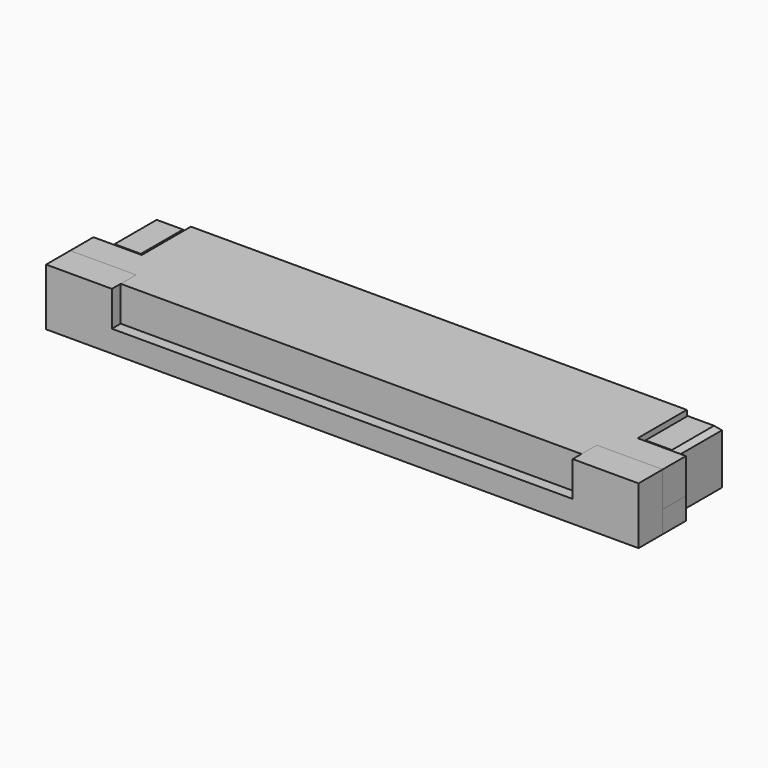
from build123d import *

# Parameters (mm, degrees)
F1_DEPTH   = 1
F2_DEPTH   = 2.6
F0_W       = 21
F0_H       = 0.5
F3_DEPTH   = 1
F5_DEPTH   = 1.6
F0_W_2     = 1.6
F0_H_2     = 2.8
F6_DEPTH   = 2.5
F0_W_3     = 0.6
F0_H_3     = 1.37
F7_DEPTH   = 0.3
F8_SIZE    = 0.2
F8_2_SIZE  = 0.2
F8_3_SIZE  = 0.2
F8_4_SIZE  = 0.2
F8_5_SIZE  = 0.2
F8_6_SIZE  = 0.2
F8_7_SIZE  = 0.2
F8_8_SIZE  = 0.2
F8_9_SIZE  = 0.2
F8_10_SIZE = 0.2
F8_11_SIZE = 0.2
F8_12_SIZE = 0.2
F8_13_SIZE = 0.2
F8_14_SIZE = 0.2
F8_15_SIZE = 0.2
F8_16_SIZE = 0.2
F8_17_SIZE = 0.2
F8_18_SIZE = 0.2
F8_19_SIZE = 0.2
F8_20_SIZE = 0.2
F9_SIZE    = 0.2
F9_2_SIZE  = 0.2


with BuildPart() as f1:
    # F0 (on Top) → F1 (new body)
    with BuildSketch(Plane.XY):
        Polygon((-9.8, 2.75), (-11.3, 2.75), (-11.3, -0.05), (-12.9, -0.05), (-13.5, -0.05), (-13.5, -1.375), (-10.5, -1.375), (-10.5, -2.25), (10.5, -2.25), (10.5, -1.375), (13.5, -1.375), (13.5, -0.05), (12.9, -0.05), (11.3, -0.05), (11.3, 2.75), (9.8, 2.75), (9.2, 2.75), (8.8, 2.75), (8.2, 2.75), (7.8, 2.75), (7.2, 2.75), (6.8, 2.75), (6.2, 2.75), (5.8, 2.75), (5.2, 2.75), (4.8, 2.75), (4.2, 2.75), (3.8, 2.75), (3.2, 2.75), (2.8, 2.75), (2.2, 2.75), (1.8, 2.75), (1.2, 2.75), (0.8, 2.75), (0.2, 2.75), (-0.2, 2.75), (-0.8, 2.75), (-1.2, 2.75), (-1.8, 2.75), (-2.2, 2.75), (-2.8, 2.75), (-3.2, 2.75), (-3.8, 2.75), (-4.2, 2.75), (-4.8, 2.75), (-5.2, 2.75), (-5.8, 2.75), (-6.2, 2.75), (-6.8, 2.75), (-7.2, 2.75), (-7.8, 2.75), (-8.2, 2.75), (-8.8, 2.75), (-9.2, 2.75), align=None)
    extrude(amount=F1_DEPTH)


with BuildPart() as f2:
    # F0 (on Top) → F2 (new body)
    with BuildSketch(Plane.XY):
        Polygon((-10.5, -1.375), (-13.5, -1.375), (-13.5, -2.75), (-10.5, -2.75), (-10.5, -2.25), align=None)
    extrude(amount=F2_DEPTH)



with BuildPart() as f2b:
    # F0 (on Top) → F2, piece 2 (new body)
    with BuildSketch(Plane.XY):
        Polygon((10.5, -2.25), (10.5, -2.75), (13.5, -2.75), (13.5, -1.375), (10.5, -1.375), align=None)
    extrude(amount=F2_DEPTH)


with BuildPart() as f2_1:
    add(f2.part)

    add(f2b.part)  # F3 merges F2b
    # F0 (on Top) → F3 (join)
    with BuildSketch(Plane.XY):
        with Locations((0, -2.5)):
            Rectangle(F0_W, F0_H)
    extrude(amount=F3_DEPTH)


with BuildPart() as f5:
    # F5 (new): a face of the model
    f5_faces = [f1.part.faces().sort_by_distance(p)[0] for p in [
        (0, 0.2268042664, 1),
    ]]
    extrude(f5_faces, amount=F5_DEPTH)


with BuildPart() as f6:
    # F0 (on Top) → F6 (new body)
    with BuildSketch(Plane.XY):
        with Locations((-12.1, 1.35)):
            Rectangle(F0_W_2, F0_H_2)
    extrude(amount=F6_DEPTH)

    # F9
    f9_edges = [f6.edges().sort_by_distance(p)[0] for p in [
        (-12.1, 2.75, 2.5),
        (-12.9, 1.35, 2.5),
        (-11.3, 1.35, 2.5),
        (-12.1, -0.05, 2.5),
    ]]
    chamfer(f9_edges, length=F9_SIZE)


with BuildPart() as f6b:
    # F0 (on Top) → F6, piece 2 (new body)
    with BuildSketch(Plane.XY):
        with Locations((12.1, 1.35)):
            Rectangle(F0_W_2, F0_H_2)
    extrude(amount=F6_DEPTH)

    # F9#2
    f9_2_edges = [f6b.edges().sort_by_distance(p)[0] for p in [
        (12.1, 2.75, 2.5),
        (12.9, 1.35, 2.5),
        (11.3, 1.35, 2.5),
        (12.1, -0.05, 2.5),
    ]]
    chamfer(f9_2_edges, length=F9_2_SIZE)


with BuildPart() as f7:
    # F0 (on Top) → F7 (new body)
    with BuildSketch(Plane.XY):
        with Locations((-9.5, 3.435)):
            Rectangle(F0_W_3, F0_H_3)
    extrude(amount=F7_DEPTH)

    # F8
    f8_edges = [f7.edges().sort_by_distance(p)[0] for p in [
        (-9.5, 4.12, 0.3),
    ]]
    chamfer(f8_edges, length=F8_SIZE)


with BuildPart() as f7b:
    # F0 (on Top) → F7, piece 2 (new body)
    with BuildSketch(Plane.XY):
        with Locations((-8.5, 3.435)):
            Rectangle(F0_W_3, F0_H_3)
    extrude(amount=F7_DEPTH)

    # F8#2
    f8_2_edges = [f7b.edges().sort_by_distance(p)[0] for p in [
        (-8.5, 4.12, 0.3),
    ]]
    chamfer(f8_2_edges, length=F8_2_SIZE)


with BuildPart() as f7c:
    # F0 (on Top) → F7, piece 3 (new body)
    with BuildSketch(Plane.XY):
        with Locations((-7.5, 3.435)):
            Rectangle(F0_W_3, F0_H_3)
    extrude(amount=F7_DEPTH)

    # F8#3
    f8_3_edges = [f7c.edges().sort_by_distance(p)[0] for p in [
        (-7.5, 4.12, 0.3),
    ]]
    chamfer(f8_3_edges, length=F8_3_SIZE)


with BuildPart() as f7d:
    # F0 (on Top) → F7, piece 4 (new body)
    with BuildSketch(Plane.XY):
        with Locations((-6.5, 3.435)):
            Rectangle(F0_W_3, F0_H_3)
    extrude(amount=F7_DEPTH)

    # F8#4
    f8_4_edges = [f7d.edges().sort_by_distance(p)[0] for p in [
        (-6.5, 4.12, 0.3),
    ]]
    chamfer(f8_4_edges, length=F8_4_SIZE)


with BuildPart() as f7e:
    # F0 (on Top) → F7, piece 5 (new body)
    with BuildSketch(Plane.XY):
        with Locations((-5.5, 3.435)):
            Rectangle(F0_W_3, F0_H_3)
    extrude(amount=F7_DEPTH)

    # F8#5
    f8_5_edges = [f7e.edges().sort_by_distance(p)[0] for p in [
        (-5.5, 4.12, 0.3),
    ]]
    chamfer(f8_5_edges, length=F8_5_SIZE)


with BuildPart() as f7f:
    # F0 (on Top) → F7, piece 6 (new body)
    with BuildSketch(Plane.XY):
        with Locations((-4.5, 3.435)):
            Rectangle(F0_W_3, F0_H_3)
    extrude(amount=F7_DEPTH)

    # F8#6
    f8_6_edges = [f7f.edges().sort_by_distance(p)[0] for p in [
        (-4.5, 4.12, 0.3),
    ]]
    chamfer(f8_6_edges, length=F8_6_SIZE)


with BuildPart() as f7g:
    # F0 (on Top) → F7, piece 7 (new body)
    with BuildSketch(Plane.XY):
        with Locations((-3.5, 3.435)):
            Rectangle(F0_W_3, F0_H_3)
    extrude(amount=F7_DEPTH)

    # F8#7
    f8_7_edges = [f7g.edges().sort_by_distance(p)[0] for p in [
        (-3.5, 4.12, 0.3),
    ]]
    chamfer(f8_7_edges, length=F8_7_SIZE)


with BuildPart() as f7h:
    # F0 (on Top) → F7, piece 8 (new body)
    with BuildSketch(Plane.XY):
        with Locations((-2.5, 3.435)):
            Rectangle(F0_W_3, F0_H_3)
    extrude(amount=F7_DEPTH)

    # F8#8
    f8_8_edges = [f7h.edges().sort_by_distance(p)[0] for p in [
        (-2.5, 4.12, 0.3),
    ]]
    chamfer(f8_8_edges, length=F8_8_SIZE)


with BuildPart() as f7i:
    # F0 (on Top) → F7, piece 9 (new body)
    with BuildSketch(Plane.XY):
        with Locations((-1.5, 3.435)):
            Rectangle(F0_W_3, F0_H_3)
    extrude(amount=F7_DEPTH)

    # F8#9
    f8_9_edges = [f7i.edges().sort_by_distance(p)[0] for p in [
        (-1.5, 4.12, 0.3),
    ]]
    chamfer(f8_9_edges, length=F8_9_SIZE)


with BuildPart() as f7j:
    # F0 (on Top) → F7, piece 10 (new body)
    with BuildSketch(Plane.XY):
        with Locations((-0.5, 3.435)):
            Rectangle(F0_W_3, F0_H_3)
    extrude(amount=F7_DEPTH)

    # F8#10
    f8_10_edges = [f7j.edges().sort_by_distance(p)[0] for p in [
        (-0.5, 4.12, 0.3),
    ]]
    chamfer(f8_10_edges, length=F8_10_SIZE)


with BuildPart() as f7k:
    # F0 (on Top) → F7, piece 11 (new body)
    with BuildSketch(Plane.XY):
        with Locations((0.5, 3.435)):
            Rectangle(F0_W_3, F0_H_3)
    extrude(amount=F7_DEPTH)

    # F8#11
    f8_11_edges = [f7k.edges().sort_by_distance(p)[0] for p in [
        (0.5, 4.12, 0.3),
    ]]
    chamfer(f8_11_edges, length=F8_11_SIZE)


with BuildPart() as f7l:
    # F0 (on Top) → F7, piece 12 (new body)
    with BuildSketch(Plane.XY):
        with Locations((1.5, 3.435)):
            Rectangle(F0_W_3, F0_H_3)
    extrude(amount=F7_DEPTH)

    # F8#12
    f8_12_edges = [f7l.edges().sort_by_distance(p)[0] for p in [
        (1.5, 4.12, 0.3),
    ]]
    chamfer(f8_12_edges, length=F8_12_SIZE)


with BuildPart() as f7m:
    # F0 (on Top) → F7, piece 13 (new body)
    with BuildSketch(Plane.XY):
        with Locations((2.5, 3.435)):
            Rectangle(F0_W_3, F0_H_3)
    extrude(amount=F7_DEPTH)

    # F8#13
    f8_13_edges = [f7m.edges().sort_by_distance(p)[0] for p in [
        (2.5, 4.12, 0.3),
    ]]
    chamfer(f8_13_edges, length=F8_13_SIZE)


with BuildPart() as f7n:
    # F0 (on Top) → F7, piece 14 (new body)
    with BuildSketch(Plane.XY):
        with Locations((3.5, 3.435)):
            Rectangle(F0_W_3, F0_H_3)
    extrude(amount=F7_DEPTH)

    # F8#14
    f8_14_edges = [f7n.edges().sort_by_distance(p)[0] for p in [
        (3.5, 4.12, 0.3),
    ]]
    chamfer(f8_14_edges, length=F8_14_SIZE)


with BuildPart() as f7o:
    # F0 (on Top) → F7, piece 15 (new body)
    with BuildSketch(Plane.XY):
        with Locations((4.5, 3.435)):
            Rectangle(F0_W_3, F0_H_3)
    extrude(amount=F7_DEPTH)

    # F8#15
    f8_15_edges = [f7o.edges().sort_by_distance(p)[0] for p in [
        (4.5, 4.12, 0.3),
    ]]
    chamfer(f8_15_edges, length=F8_15_SIZE)


with BuildPart() as f7p:
    # F0 (on Top) → F7, piece 16 (new body)
    with BuildSketch(Plane.XY):
        with Locations((5.5, 3.435)):
            Rectangle(F0_W_3, F0_H_3)
    extrude(amount=F7_DEPTH)

    # F8#16
    f8_16_edges = [f7p.edges().sort_by_distance(p)[0] for p in [
        (5.5, 4.12, 0.3),
    ]]
    chamfer(f8_16_edges, length=F8_16_SIZE)


with BuildPart() as f7q:
    # F0 (on Top) → F7, piece 17 (new body)
    with BuildSketch(Plane.XY):
        with Locations((6.5, 3.435)):
            Rectangle(F0_W_3, F0_H_3)
    extrude(amount=F7_DEPTH)

    # F8#17
    f8_17_edges = [f7q.edges().sort_by_distance(p)[0] for p in [
        (6.5, 4.12, 0.3),
    ]]
    chamfer(f8_17_edges, length=F8_17_SIZE)


with BuildPart() as f7r:
    # F0 (on Top) → F7, piece 18 (new body)
    with BuildSketch(Plane.XY):
        with Locations((7.5, 3.435)):
            Rectangle(F0_W_3, F0_H_3)
    extrude(amount=F7_DEPTH)

    # F8#18
    f8_18_edges = [f7r.edges().sort_by_distance(p)[0] for p in [
        (7.5, 4.12, 0.3),
    ]]
    chamfer(f8_18_edges, length=F8_18_SIZE)


with BuildPart() as f7s:
    # F0 (on Top) → F7, piece 19 (new body)
    with BuildSketch(Plane.XY):
        with Locations((8.5, 3.435)):
            Rectangle(F0_W_3, F0_H_3)
    extrude(amount=F7_DEPTH)

    # F8#19
    f8_19_edges = [f7s.edges().sort_by_distance(p)[0] for p in [
        (8.5, 4.12, 0.3),
    ]]
    chamfer(f8_19_edges, length=F8_19_SIZE)


with BuildPart() as f7t:
    # F0 (on Top) → F7, piece 20 (new body)
    with BuildSketch(Plane.XY):
        with Locations((9.5, 3.435)):
            Rectangle(F0_W_3, F0_H_3)
    extrude(amount=F7_DEPTH)

    # F8#20
    f8_20_edges = [f7t.edges().sort_by_distance(p)[0] for p in [
        (9.5, 4.12, 0.3),
    ]]
    chamfer(f8_20_edges, length=F8_20_SIZE)


solid = Compound([f1.part, f2_1.part, f5.part, f6.part, f6b.part, f7.part, f7b.part, f7c.part, f7d.part, f7e.part, f7f.part, f7g.part, f7h.part, f7i.part, f7j.part, f7k.part, f7l.part, f7m.part, f7n.part, f7o.part, f7p.part, f7q.part, f7r.part, f7s.part, f7t.part])
